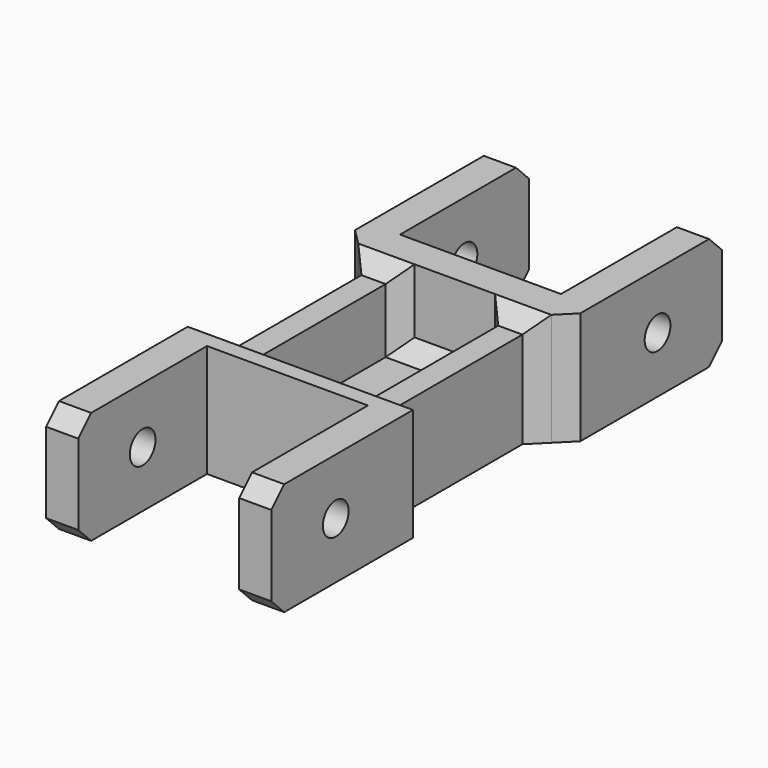
from build123d import *

# Parameters (mm, degrees)
F0_W            = 20
F0_H            = 22
F0_H_2          = 4
F0_H_3          = 20.4
F1_DEPTH        = 2
F2_DEPTH        = 10
F3_R            = 2.2
F4_DEPTH        = 30
F5_W            = 20
F5_H            = 12
F5_R            = 2.6
F7_DEPTH        = 4
F6_W            = 20
F6_H            = 12
F6_R            = 2.6
F8_DEPTH        = 4
F9_T1_DEPTH     = 25
F9_T3_DEPTH     = 57.4
F9_T5_DEPTH     = 16
F9_T7_DEPTH     = 48.4
F9_T9_DEPTH     = 2
F9_T11_DEPTH    = 20
F9_T13_DEPTH    = 7
F9_T15_DEPTH    = 25
F9_T17_DEPTH    = 14
F9_T19_DEPTH    = 27
F9_T21_DEPTH    = 14
F9_T23_DEPTH    = 30
F9_T25_DEPTH    = 7
F9_T27_DEPTH    = 8
F9_S31_W        = 2
F9_S31_H        = 2
F9_T32_DEPTH    = 2
F9_S37_W        = 2
F9_S37_H        = 2
F9_T38_DEPTH    = 2
F9_S43_W        = 2
F9_S43_H        = 2
F9_T44_DEPTH    = 2
F9_S49_W        = 2
F9_S49_H        = 2
F9_T50_DEPTH    = 2
F9_S55_W        = 2
F9_S55_H        = 2
F9_T56_DEPTH    = 2
F9_S61_W        = 2
F9_S61_H        = 2
F9_T62_DEPTH    = 2
F9_S67_W        = 2
F9_S67_H        = 2
F9_T68_DEPTH    = 2
F9_S73_W        = 2
F9_S73_H        = 2
F9_T74_DEPTH    = 2
F9_T81_DEPTH    = 30
F9_T85_DEPTH    = 30
F9_T92_DEPTH    = 7
F9_T96_DEPTH    = 53.4
F9_T103_DEPTH   = 30
F9_T107_DEPTH   = 30
F9_S1_T1_DEPTH  = 7
F9_S1_T3_DEPTH  = 30
F9_S1_T5_DEPTH  = 16
F9_S1_T7_DEPTH  = 8
F9_S1_S11_W     = 2
F9_S1_S11_H     = 2
F9_S1_T12_DEPTH = 2
F9_S1_S17_W     = 2
F9_S1_S17_H     = 2
F9_S1_T18_DEPTH = 2
F9_S1_S23_W     = 2
F9_S1_S23_H     = 2
F9_S1_T24_DEPTH = 2
F9_S1_S29_W     = 2
F9_S1_S29_H     = 2
F9_S1_T30_DEPTH = 2
F10_W           = 20
F10_H           = 30
F11_DEPTH       = 4
F12_W           = 20
F12_H           = 4
F13_DEPTH       = 10
F16_DEPTH       = 4
F17_DEPTH       = 4
F19_W           = 4
F19_H           = 14
F20_DEPTH       = 20
F18_W           = 4
F18_H           = 14
F21_DEPTH       = 20
F22_W           = 22
F22_H           = 8
F23_DEPTH       = 3
F24_W           = 22
F24_H           = 8
F25_DEPTH       = 3
F26_R           = 2
F27_R           = 2
F28_DEPTH       = 28.3421242009
F29_SIZE        = 1.99999


# Not quite as in the source:
# - a fillet or chamfer that OpenCascade refuses, or shapes differently, is made with other operations: its cross-section is extruded or revolved along the edge and cut away or added
# - a fillet or chamfer is up to 0.001 mm smaller than in the source, because OpenCascade refuses the exact size
# - a feature names something its author has since deleted; it is built from what else it names


with BuildPart() as f1:
    # F0 (on Top) → F1 (new body)
    with BuildSketch(Plane.XY):
        with Locations((-44.4073281825, 48.6883277684)):
            Rectangle(F0_W, F0_H)
        with Locations((-44.4073281825, 61.6883277684)):
            Rectangle(F0_W, F0_H_2)
        with Locations((-44.4073281825, 35.6883277684)):
            Rectangle(F0_W, F0_H_2)
        with Locations((-44.4073281825, 23.4883277684)):
            Rectangle(F0_W, F0_H_3)
        with Locations((-44.4073281825, 11.2883277684)):
            Rectangle(F0_W, F0_H_2)
    extrude(amount=-F1_DEPTH)

    # F0 (on Top) → F2 (join)
    with BuildSketch(Plane.XY):
        with Locations((-44.4073281825, 35.6883277684)):
            Rectangle(F0_W, F0_H_2)
        with Locations((-44.4073281825, 61.6883277684)):
            Rectangle(F0_W, F0_H_2)
        with Locations((-44.4073281825, 11.2883277684)):
            Rectangle(F0_W, F0_H_2)
    extrude(amount=F2_DEPTH)

    # F3 (on face) → F4 (cut)
    with BuildSketch(Plane.XZ.offset(-9.2883277684)):
        with Locations((-44.4073281825, 5.5)):
            Circle(F3_R)
    extrude(amount=-F4_DEPTH, mode=Mode.SUBTRACT)

    # F5 (on face) → F7 (join)
    with BuildSketch(Plane(origin=(-54.4073281825, 0, 0), x_dir=(0, -1, 0), z_dir=(-1, 0, 0))):
        with Locations((-73.6883277684, 4)):
            Rectangle(F5_W, F5_H)
        with Locations((-73.6883277684, 4)):
            Circle(F5_R, mode=Mode.SUBTRACT)
    extrude(amount=F7_DEPTH)

    # F6 (on face) → F8 (join)
    with BuildSketch(Plane.YZ.offset(-34.4073281825)):
        with Locations((73.6883277684, 4)):
            Rectangle(F6_W, F6_H)
        with Locations((73.6883277684, 4)):
            Circle(F6_R, mode=Mode.SUBTRACT)
        Polygon((63.6883277684, 10), (59.6883277684, 10), (59.6883277684, 0), (59.6883277684, -2), (63.6883277684, -2), align=None)
    extrude(amount=F8_DEPTH)

    # F9: fillet of radius 2 on 26 edges, made by hand

    # F9_s2 → F9_t1 (cut)
    with BuildSketch(Plane.YZ.offset(-59.4073281825)):
        with BuildLine():
            ThreePointArc((63.6883277684, 0), (63.1025413308, -1.4142135624), (61.6883277684, -2))
            Line((61.6883277684, -2), (63.6883277684, -2))
            Line((63.6883277684, -2), (63.6883277684, 0))
        make_face()
        with BuildLine():
            ThreePointArc((63.6883277684, 8), (63.1025413308, 9.4142135624), (61.6883277684, 10))
            Line((61.6883277684, 10), (63.6883277684, 10))
            Line((63.6883277684, 10), (63.6883277684, 8))
        make_face()
    extrude(amount=F9_T1_DEPTH, mode=Mode.SUBTRACT)

    # F9_s4 → F9_t3 (cut)
    with BuildSketch(Plane.XZ.offset(-68.6883277684)):
        with BuildLine():
            ThreePointArc((-54.4073281825, 0), (-53.8215417448, -1.4142135624), (-52.4073281825, -2))
            Line((-52.4073281825, -2), (-54.4073281825, -2))
            Line((-54.4073281825, -2), (-54.4073281825, 0))
        make_face()
    extrude(amount=F9_T3_DEPTH, mode=Mode.SUBTRACT)

    # F9_s6 → F9_t5 (cut)
    with BuildSketch(Plane.YZ.offset(-52.4073281825)):
        with BuildLine():
            ThreePointArc((9.2883277684, 0), (9.8741142061, -1.4142135624), (11.2883277684, -2))
            Line((11.2883277684, -2), (9.2883277684, -2))
            Line((9.2883277684, -2), (9.2883277684, 0))
        make_face()
        with BuildLine():
            ThreePointArc((9.2883277684, 8), (9.8741142061, 9.4142135624), (11.2883277684, 10))
            Line((11.2883277684, 10), (9.2883277684, 10))
            Line((9.2883277684, 10), (9.2883277684, 8))
        make_face()
    extrude(amount=F9_T5_DEPTH, mode=Mode.SUBTRACT)

    # F9_s8 → F9_t7 (cut)
    with BuildSketch(Plane.XZ.offset(-59.6883277684)):
        with BuildLine():
            ThreePointArc((-34.4073281825, 0), (-34.9931146201, -1.4142135624), (-36.4073281825, -2))
            Line((-36.4073281825, -2), (-34.4073281825, -2))
            Line((-34.4073281825, -2), (-34.4073281825, 0))
        make_face()
    extrude(amount=F9_T7_DEPTH, mode=Mode.SUBTRACT)

    # F9_s10 → F9_t9 (cut)
    with BuildSketch(Plane.YZ.offset(-34.4073281825)):
        with BuildLine():
            ThreePointArc((59.6883277684, 0), (60.2741142061, -1.4142135624), (61.6883277684, -2))
            Line((61.6883277684, -2), (59.6883277684, -2))
            Line((59.6883277684, -2), (59.6883277684, 0))
        make_face()
    extrude(amount=F9_T9_DEPTH, mode=Mode.SUBTRACT)

    # F9_s12 → F9_t11 (cut)
    with BuildSketch(Plane.XZ.offset(-81.6883277684)):
        with BuildLine():
            ThreePointArc((-30.4073281825, 0), (-30.9931146201, -1.4142135624), (-32.4073281825, -2))
            Line((-32.4073281825, -2), (-30.4073281825, -2))
            Line((-30.4073281825, -2), (-30.4073281825, 0))
        make_face()
        with BuildLine():
            ThreePointArc((-30.4073281825, 8), (-30.9931146201, 9.4142135624), (-32.4073281825, 10))
            Line((-32.4073281825, 10), (-30.4073281825, 10))
            Line((-30.4073281825, 10), (-30.4073281825, 8))
        make_face()
    extrude(amount=F9_T11_DEPTH, mode=Mode.SUBTRACT)

    # F9_s14 → F9_t13 (cut)
    with BuildSketch(Plane.YZ.offset(-39.4073281825)):
        with BuildLine():
            ThreePointArc((83.6883277684, 0), (83.1025413308, -1.4142135624), (81.6883277684, -2))
            Line((81.6883277684, -2), (83.6883277684, -2))
            Line((83.6883277684, -2), (83.6883277684, 0))
        make_face()
        with BuildLine():
            ThreePointArc((83.6883277684, 8), (83.1025413308, 9.4142135624), (81.6883277684, 10))
            Line((81.6883277684, 10), (83.6883277684, 10))
            Line((83.6883277684, 10), (83.6883277684, 8))
        make_face()
    extrude(amount=F9_T13_DEPTH, mode=Mode.SUBTRACT)

    # F9_s16 → F9_t15 (cut)
    with BuildSketch(Plane.XZ.offset(-88.6883277684)):
        with BuildLine():
            ThreePointArc((-34.4073281825, 0), (-33.8215417448, -1.4142135624), (-32.4073281825, -2))
            Line((-32.4073281825, -2), (-34.4073281825, -2))
            Line((-34.4073281825, -2), (-34.4073281825, 0))
        make_face()
        with BuildLine():
            ThreePointArc((-34.4073281825, 8), (-33.8215417448, 9.4142135624), (-32.4073281825, 10))
            Line((-32.4073281825, 10), (-34.4073281825, 10))
            Line((-34.4073281825, 10), (-34.4073281825, 8))
        make_face()
    extrude(amount=F9_T15_DEPTH, mode=Mode.SUBTRACT)

    # F9_s18 → F9_t17 (cut)
    with BuildSketch(Plane.XZ.offset(-68.6883277684)):
        with BuildLine():
            ThreePointArc((-52.4073281825, 10), (-53.8215417448, 9.4142135624), (-54.4073281825, 8))
            Line((-54.4073281825, 8), (-54.4073281825, 10))
            Line((-54.4073281825, 10), (-52.4073281825, 10))
        make_face()
    extrude(amount=F9_T17_DEPTH, mode=Mode.SUBTRACT)

    # F9_s20 → F9_t19 (cut)
    with BuildSketch(Plane.YZ.offset(-59.4073281825)):
        with BuildLine():
            ThreePointArc((59.6883277684, 8), (60.2741142061, 9.4142135624), (61.6883277684, 10))
            Line((61.6883277684, 10), (59.6883277684, 10))
            Line((59.6883277684, 10), (59.6883277684, 8))
        make_face()
    extrude(amount=F9_T19_DEPTH, mode=Mode.SUBTRACT)

    # F9_s22 → F9_t21 (cut)
    with BuildSketch(Plane.XZ.offset(-42.6883277684)):
        with BuildLine():
            ThreePointArc((-52.4073281825, 10), (-53.8215417448, 9.4142135624), (-54.4073281825, 8))
            Line((-54.4073281825, 8), (-54.4073281825, 10))
            Line((-54.4073281825, 10), (-52.4073281825, 10))
        make_face()
        with BuildLine():
            ThreePointArc((-36.4073281825, 10), (-34.9931146201, 9.4142135624), (-34.4073281825, 8))
            Line((-34.4073281825, 8), (-34.4073281825, 10))
            Line((-34.4073281825, 10), (-36.4073281825, 10))
        make_face()
    extrude(amount=F9_T21_DEPTH, mode=Mode.SUBTRACT)

    # F9_s24 → F9_t23 (cut)
    with BuildSketch(Plane.YZ.offset(-59.4073281825)):
        with BuildLine():
            ThreePointArc((33.6883277684, 8), (34.2741142061, 9.4142135624), (35.6883277684, 10))
            Line((35.6883277684, 10), (33.6883277684, 10))
            Line((33.6883277684, 10), (33.6883277684, 8))
        make_face()
        with BuildLine():
            ThreePointArc((37.6883277684, 8), (37.1025413308, 9.4142135624), (35.6883277684, 10))
            Line((35.6883277684, 10), (37.6883277684, 10))
            Line((37.6883277684, 10), (37.6883277684, 8))
        make_face()
        with BuildLine():
            ThreePointArc((13.2883277684, 8), (12.7025413308, 9.4142135624), (11.2883277684, 10))
            Line((11.2883277684, 10), (13.2883277684, 10))
            Line((13.2883277684, 10), (13.2883277684, 8))
        make_face()
    extrude(amount=F9_T23_DEPTH, mode=Mode.SUBTRACT)

    # F9_s26 → F9_t25 (cut)
    with BuildSketch(Plane.XZ.offset(-18.2883277684)):
        with BuildLine():
            ThreePointArc((-36.4073281825, 10), (-34.9931146201, 9.4142135624), (-34.4073281825, 8))
            Line((-34.4073281825, 8), (-34.4073281825, 10))
            Line((-34.4073281825, 10), (-36.4073281825, 10))
        make_face()
        with BuildLine():
            ThreePointArc((-52.4073281825, 10), (-53.8215417448, 9.4142135624), (-54.4073281825, 8))
            Line((-54.4073281825, 8), (-54.4073281825, 10))
            Line((-54.4073281825, 10), (-52.4073281825, 10))
        make_face()
    extrude(amount=F9_T25_DEPTH, mode=Mode.SUBTRACT)

    # F9_s28 → F9_t27 (cut)
    with BuildSketch(Plane.XY):
        with BuildLine():
            ThreePointArc((-36.4073281825, 9.2883277684), (-34.9931146201, 9.8741142061), (-34.4073281825, 11.2883277684))
            Line((-34.4073281825, 11.2883277684), (-34.4073281825, 9.2883277684))
            Line((-34.4073281825, 9.2883277684), (-36.4073281825, 9.2883277684))
        make_face()
        with BuildLine():
            ThreePointArc((-52.4073281825, 9.2883277684), (-53.8215417448, 9.8741142061), (-54.4073281825, 11.2883277684))
            Line((-54.4073281825, 11.2883277684), (-54.4073281825, 9.2883277684))
            Line((-54.4073281825, 9.2883277684), (-52.4073281825, 9.2883277684))
        make_face()
        with BuildLine():
            ThreePointArc((-30.4073281825, 61.6883277684), (-30.9931146201, 60.2741142061), (-32.4073281825, 59.6883277684))
            Line((-32.4073281825, 59.6883277684), (-30.4073281825, 59.6883277684))
            Line((-30.4073281825, 59.6883277684), (-30.4073281825, 61.6883277684))
        make_face()
        with BuildLine():
            ThreePointArc((-30.4073281825, 81.6883277684), (-30.9931146201, 83.1025413308), (-32.4073281825, 83.6883277684))
            Line((-32.4073281825, 83.6883277684), (-30.4073281825, 83.6883277684))
            Line((-30.4073281825, 83.6883277684), (-30.4073281825, 81.6883277684))
        make_face()
    extrude(amount=F9_T27_DEPTH, mode=Mode.SUBTRACT)


with BuildPart() as f9_tool30:
    # F9_s31 → F9_t32 (new body)
    with BuildSketch(Plane.YZ.offset(-52.4073281825)):
        with Locations((10.2883277684, -1)):
            Rectangle(F9_S31_W, F9_S31_H)
    extrude(amount=-F9_T32_DEPTH)

    # F9_s33 → F9_t34 (revolve, cut)
    with BuildSketch(Plane(origin=(-52.4073281825, 11.2883277684, 0), x_dir=(0, 0.7071067812, 0.7071067812), z_dir=(0, -0.7071067812, 0.7071067812))):
        with BuildLine():
            ThreePointArc((0, -2), (2, 0), (0, 2))
            Line((0, 2), (0, -2))
        make_face()
    revolve(axis=Axis((-52.4073281825, 11.2883277684, 0), (-1, 0, 0)), mode=Mode.SUBTRACT)


with BuildPart() as f1_1:
    add(f1.part)

    # F9_t29: cut F9_tool30
    add(f9_tool30.part, mode=Mode.SUBTRACT)


with BuildPart() as f9_tool36:
    # F9_s37 → F9_t38 (new body)
    with BuildSketch(Plane.XY):
        with Locations((-35.4073281825, 10.2883277684)):
            Rectangle(F9_S37_W, F9_S37_H)
    extrude(amount=-F9_T38_DEPTH)

    # F9_s39 → F9_t40 (revolve, cut)
    with BuildSketch(Plane(origin=(-36.4073281825, 11.2883277684, 0), x_dir=(-0.7071067812, 0.7071067812, 0), z_dir=(-0.7071067812, -0.7071067812, 0))):
        with BuildLine():
            ThreePointArc((0, -2), (2, 0), (0, 2))
            Line((0, 2), (0, -2))
        make_face()
    revolve(axis=Axis((-36.4073281825, 11.2883277684, 0), (0, 0, -1)), mode=Mode.SUBTRACT)


with BuildPart() as f1_2:
    add(f1_1.part)

    # F9_t35: cut F9_tool36
    add(f9_tool36.part, mode=Mode.SUBTRACT)


with BuildPart() as f9_tool42:
    # F9_s43 → F9_t44 (new body)
    with BuildSketch(Plane.YZ.offset(-32.4073281825)):
        with Locations((60.6883277684, -1)):
            Rectangle(F9_S43_W, F9_S43_H)
    extrude(amount=F9_T44_DEPTH)

    # F9_s45 → F9_t46 (revolve, cut)
    with BuildSketch(Plane(origin=(-32.4073281825, 61.6883277684, 0), x_dir=(0, 0.7071067812, 0.7071067812), z_dir=(0, 0.7071067812, -0.7071067812))):
        with BuildLine():
            ThreePointArc((0, -2), (2, 0), (0, 2))
            Line((0, 2), (0, -2))
        make_face()
    revolve(axis=Axis((-32.4073281825, 61.6883277684, 0), (1, 0, 0)), mode=Mode.SUBTRACT)


with BuildPart() as f1_3:
    add(f1_2.part)

    # F9_t41: cut F9_tool42
    add(f9_tool42.part, mode=Mode.SUBTRACT)


with BuildPart() as f9_tool48:
    # F9_s49 → F9_t50 (new body)
    with BuildSketch(Plane.XY):
        with Locations((-31.4073281825, 82.6883277684)):
            Rectangle(F9_S49_W, F9_S49_H)
    extrude(amount=-F9_T50_DEPTH)

    # F9_s51 → F9_t52 (revolve, cut)
    with BuildSketch(Plane(origin=(-32.4073281825, 81.6883277684, 0), x_dir=(-0.7071067812, -0.7071067812, 0), z_dir=(0.7071067812, -0.7071067812, 0))):
        with BuildLine():
            ThreePointArc((0, -2), (2, 0), (0, 2))
            Line((0, 2), (0, -2))
        make_face()
    revolve(axis=Axis((-32.4073281825, 81.6883277684, 0), (0, 0, -1)), mode=Mode.SUBTRACT)


with BuildPart() as f1_4:
    add(f1_3.part)

    # F9_t47: cut F9_tool48
    add(f9_tool48.part, mode=Mode.SUBTRACT)


with BuildPart() as f9_tool54:
    # F9_s55 → F9_t56 (new body)
    with BuildSketch(Plane.XY.offset(8)):
        with Locations((-31.4073281825, 60.6883277684)):
            Rectangle(F9_S55_W, F9_S55_H)
    extrude(amount=F9_T56_DEPTH)

    # F9_s57 → F9_t58 (revolve, cut)
    with BuildSketch(Plane(origin=(-32.4073281825, 61.6883277684, 8), x_dir=(-0.7071067812, 0.7071067812, 0), z_dir=(0.7071067812, 0.7071067812, 0))):
        with BuildLine():
            ThreePointArc((0, -2), (2, 0), (0, 2))
            Line((0, 2), (0, -2))
        make_face()
    revolve(axis=Axis((-32.4073281825, 61.6883277684, 8), (0, 0, 1)), mode=Mode.SUBTRACT)


with BuildPart() as f1_5:
    add(f1_4.part)

    # F9_t53: cut F9_tool54
    add(f9_tool54.part, mode=Mode.SUBTRACT)


with BuildPart() as f9_tool60:
    # F9_s61 → F9_t62 (new body)
    with BuildSketch(Plane.XZ.offset(-81.6883277684)):
        with Locations((-31.4073281825, 9)):
            Rectangle(F9_S61_W, F9_S61_H)
    extrude(amount=-F9_T62_DEPTH)

    # F9_s63 → F9_t64 (revolve, cut)
    with BuildSketch(Plane(origin=(-32.4073281825, 81.6883277684, 8), x_dir=(-0.7071067812, 0, -0.7071067812), z_dir=(0.7071067812, 0, -0.7071067812))):
        with BuildLine():
            ThreePointArc((0, -2), (2, 0), (0, 2))
            Line((0, 2), (0, -2))
        make_face()
    revolve(axis=Axis((-32.4073281825, 81.6883277684, 8), (0, 1, 0)), mode=Mode.SUBTRACT)


with BuildPart() as f1_6:
    add(f1_5.part)

    # F9_t59: cut F9_tool60
    add(f9_tool60.part, mode=Mode.SUBTRACT)


with BuildPart() as f9_tool66:
    # F9_s67 → F9_t68 (new body)
    with BuildSketch(Plane.XZ.offset(-11.2883277684)):
        with Locations((-35.4073281825, 9)):
            Rectangle(F9_S67_W, F9_S67_H)
    extrude(amount=F9_T68_DEPTH)

    # F9_s69 → F9_t70 (revolve, cut)
    with BuildSketch(Plane(origin=(-36.4073281825, 11.2883277684, 8), x_dir=(-0.7071067812, 0, -0.7071067812), z_dir=(-0.7071067812, 0, 0.7071067812))):
        with BuildLine():
            ThreePointArc((0, -2), (2, 0), (0, 2))
            Line((0, 2), (0, -2))
        make_face()
    revolve(axis=Axis((-36.4073281825, 11.2883277684, 8), (0, -1, 0)), mode=Mode.SUBTRACT)


with BuildPart() as f1_7:
    add(f1_6.part)

    # F9_t65: cut F9_tool66
    add(f9_tool66.part, mode=Mode.SUBTRACT)


with BuildPart() as f9_tool72:
    # F9_s73 → F9_t74 (new body)
    with BuildSketch(Plane.YZ.offset(-52.4073281825)):
        with Locations((10.2883277684, 9)):
            Rectangle(F9_S73_W, F9_S73_H)
    extrude(amount=-F9_T74_DEPTH)

    # F9_s75 → F9_t76 (revolve, cut)
    with BuildSketch(Plane(origin=(-52.4073281825, 11.2883277684, 8), x_dir=(0, 0.7071067812, -0.7071067812), z_dir=(0, 0.7071067812, 0.7071067812))):
        with BuildLine():
            ThreePointArc((0, -2), (2, 0), (0, 2))
            Line((0, 2), (0, -2))
        make_face()
    revolve(axis=Axis((-52.4073281825, 11.2883277684, 8), (-1, 0, 0)), mode=Mode.SUBTRACT)


with BuildPart() as f1_8:
    add(f1_7.part)

    # F9_t71: cut F9_tool72
    add(f9_tool72.part, mode=Mode.SUBTRACT)


with BuildPart() as f9_tool79:
    # F9_s80 → F9_t81 (new body)
    with BuildSketch(Plane.YZ.offset(-29.4073281825)):
        with BuildLine():
            ThreePointArc((63.6883277684, 0), (63.1025413308, -1.4142135624), (61.6883277684, -2))
            Line((61.6883277684, -2), (63.6883277684, -2))
            Line((63.6883277684, -2), (63.6883277684, 0))
        make_face()
    extrude(amount=-F9_T81_DEPTH)

    split(bisect_by=Plane.YZ.offset(-34.4073281825), keep=Keep.TOP)


with BuildPart() as f9_tool83:
    # F9_s84 → F9_t85 (new body)
    with BuildSketch(Plane.XZ.offset(-58.6883277684)):
        with BuildLine():
            ThreePointArc((-34.4073281825, 0), (-33.8215417448, -1.4142135624), (-32.4073281825, -2))
            Line((-32.4073281825, -2), (-34.4073281825, -2))
            Line((-34.4073281825, -2), (-34.4073281825, 0))
        make_face()
    extrude(amount=-F9_T85_DEPTH)

    split(bisect_by=Plane.XZ.offset(-63.6883277684), keep=Keep.TOP)


with BuildPart() as f9_tool79_1:
    add(f9_tool79.part)

    # F9_t87: intersect F9_tool83
    add(f9_tool83.part, mode=Mode.INTERSECT)


with BuildPart() as f1_9:
    add(f1_8.part)

    # F9_t77: cut F9_tool79
    add(f9_tool79_1.part, mode=Mode.SUBTRACT)


with BuildPart() as f9_tool90:
    # F9_s91 → F9_t92 (new body)
    with BuildSketch(Plane.YZ.offset(-39.4073281825)):
        with BuildLine():
            ThreePointArc((59.6883277684, 0), (60.2741142061, -1.4142135624), (61.6883277684, -2))
            Line((61.6883277684, -2), (59.6883277684, -2))
            Line((59.6883277684, -2), (59.6883277684, 0))
        make_face()
    extrude(amount=F9_T92_DEPTH)

    split(bisect_by=Plane.YZ.offset(-34.4073281825), keep=Keep.BOTTOM)


with BuildPart() as f9_tool94:
    # F9_s95 → F9_t96 (new body)
    with BuildSketch(Plane.XZ.offset(-11.2883277684)):
        with BuildLine():
            ThreePointArc((-34.4073281825, 0), (-34.9931146201, -1.4142135624), (-36.4073281825, -2))
            Line((-36.4073281825, -2), (-34.4073281825, -2))
            Line((-34.4073281825, -2), (-34.4073281825, 0))
        make_face()
    extrude(amount=-F9_T96_DEPTH)

    split(bisect_by=Plane.XZ.offset(-59.6883277684), keep=Keep.BOTTOM)


with BuildPart() as f9_tool90_1:
    add(f9_tool90.part)

    # F9_t98: intersect F9_tool94
    add(f9_tool94.part, mode=Mode.INTERSECT)


with BuildPart() as f1_10:
    add(f1_9.part)

    # F9_t88: cut F9_tool90
    add(f9_tool90_1.part, mode=Mode.SUBTRACT)


with BuildPart() as f9_tool101:
    # F9_s102 → F9_t103 (new body)
    with BuildSketch(Plane.YZ.offset(-29.4073281825)):
        with BuildLine():
            ThreePointArc((63.6883277684, 8), (63.1025413308, 9.4142135624), (61.6883277684, 10))
            Line((61.6883277684, 10), (63.6883277684, 10))
            Line((63.6883277684, 10), (63.6883277684, 8))
        make_face()
    extrude(amount=-F9_T103_DEPTH)

    split(bisect_by=Plane.YZ.offset(-34.4073281825), keep=Keep.TOP)


with BuildPart() as f9_tool105:
    # F9_s106 → F9_t107 (new body)
    with BuildSketch(Plane.XZ.offset(-88.6883277684)):
        with BuildLine():
            ThreePointArc((-34.4073281825, 8), (-33.8215417448, 9.4142135624), (-32.4073281825, 10))
            Line((-32.4073281825, 10), (-34.4073281825, 10))
            Line((-34.4073281825, 10), (-34.4073281825, 8))
        make_face()
    extrude(amount=F9_T107_DEPTH)

    split(bisect_by=Plane.XZ.offset(-63.6883277684), keep=Keep.TOP)


with BuildPart() as f9_tool101_1:
    add(f9_tool101.part)

    # F9_t109: intersect F9_tool105
    add(f9_tool105.part, mode=Mode.INTERSECT)


with BuildPart() as f1_11:
    add(f1_10.part)

    # F9_t99: cut F9_tool101
    add(f9_tool101_1.part, mode=Mode.SUBTRACT)

    # F9#s1: fillet of radius 2 on 10 edges, made by hand

    # F9_s1_s2 → F9_s1_t1 (cut)
    with BuildSketch(Plane.YZ.offset(-56.4073281825)):
        with BuildLine():
            ThreePointArc((83.6883277684, 0), (83.1025413308, -1.4142135624), (81.6883277684, -2))
            Line((81.6883277684, -2), (83.6883277684, -2))
            Line((83.6883277684, -2), (83.6883277684, 0))
        make_face()
        with BuildLine():
            ThreePointArc((63.6883277684, 0), (64.2741142061, -1.4142135624), (65.6883277684, -2))
            Line((65.6883277684, -2), (63.6883277684, -2))
            Line((63.6883277684, -2), (63.6883277684, 0))
        make_face()
        with BuildLine():
            ThreePointArc((63.6883277684, 8), (64.2741142061, 9.4142135624), (65.6883277684, 10))
            Line((65.6883277684, 10), (63.6883277684, 10))
            Line((63.6883277684, 10), (63.6883277684, 8))
        make_face()
        with BuildLine():
            ThreePointArc((81.6883277684, 10), (83.1025413308, 9.4142135624), (83.6883277684, 8))
            Line((83.6883277684, 8), (83.6883277684, 10))
            Line((83.6883277684, 10), (81.6883277684, 10))
        make_face()
    extrude(amount=F9_S1_T1_DEPTH, mode=Mode.SUBTRACT)

    # F9_s1_s4 → F9_s1_t3 (cut)
    with BuildSketch(Plane.XZ.offset(-88.6883277684)):
        with BuildLine():
            ThreePointArc((-56.4073281825, -2), (-54.9931146201, -1.4142135624), (-54.4073281825, 0))
            Line((-54.4073281825, 0), (-54.4073281825, -2))
            Line((-54.4073281825, -2), (-56.4073281825, -2))
        make_face()
        with BuildLine():
            ThreePointArc((-56.4073281825, 10), (-54.9931146201, 9.4142135624), (-54.4073281825, 8))
            Line((-54.4073281825, 8), (-54.4073281825, 10))
            Line((-54.4073281825, 10), (-56.4073281825, 10))
        make_face()
    extrude(amount=F9_S1_T3_DEPTH, mode=Mode.SUBTRACT)

    # F9_s1_s6 → F9_s1_t5 (cut)
    with BuildSketch(Plane.XZ.offset(-81.6883277684)):
        with BuildLine():
            ThreePointArc((-58.4073281825, 0), (-57.8215417448, -1.4142135624), (-56.4073281825, -2))
            Line((-56.4073281825, -2), (-58.4073281825, -2))
            Line((-58.4073281825, -2), (-58.4073281825, 0))
        make_face()
        with BuildLine():
            ThreePointArc((-56.4073281825, 10), (-57.8215417448, 9.4142135624), (-58.4073281825, 8))
            Line((-58.4073281825, 8), (-58.4073281825, 10))
            Line((-58.4073281825, 10), (-56.4073281825, 10))
        make_face()
    extrude(amount=F9_S1_T5_DEPTH, mode=Mode.SUBTRACT)

    # F9_s1_s8 → F9_s1_t7 (cut)
    with BuildSketch(Plane.XY):
        with BuildLine():
            ThreePointArc((-56.4073281825, 63.6883277684), (-57.8215417448, 64.2741142061), (-58.4073281825, 65.6883277684))
            Line((-58.4073281825, 65.6883277684), (-58.4073281825, 63.6883277684))
            Line((-58.4073281825, 63.6883277684), (-56.4073281825, 63.6883277684))
        make_face()
        with BuildLine():
            ThreePointArc((-56.4073281825, 83.6883277684), (-57.8215417448, 83.1025413308), (-58.4073281825, 81.6883277684))
            Line((-58.4073281825, 81.6883277684), (-58.4073281825, 83.6883277684))
            Line((-58.4073281825, 83.6883277684), (-56.4073281825, 83.6883277684))
        make_face()
    extrude(amount=F9_S1_T7_DEPTH, mode=Mode.SUBTRACT)


with BuildPart() as f9_s1_tool10:
    # F9_s1_s11 → F9_s1_t12 (new body)
    with BuildSketch(Plane.XZ.offset(-81.6883277684)):
        with Locations((-57.4073281825, -1)):
            Rectangle(F9_S1_S11_W, F9_S1_S11_H)
    extrude(amount=-F9_S1_T12_DEPTH)

    # F9_s1_s13 → F9_s1_t14 (revolve, cut)
    with BuildSketch(Plane(origin=(-56.4073281825, 81.6883277684, 0), x_dir=(0.7071067812, 0, 0.7071067812), z_dir=(-0.7071067812, 0, 0.7071067812))):
        with BuildLine():
            ThreePointArc((0, -2), (2, 0), (0, 2))
            Line((0, 2), (0, -2))
        make_face()
    revolve(axis=Axis((-56.4073281825, 81.6883277684, 0), (0, 1, 0)), mode=Mode.SUBTRACT)


with BuildPart() as f1_12:
    add(f1_11.part)

    # F9_s1_t9: cut F9_s1_tool10
    add(f9_s1_tool10.part, mode=Mode.SUBTRACT)


with BuildPart() as f9_s1_tool16:
    # F9_s1_s17 → F9_s1_t18 (new body)
    with BuildSketch(Plane.XZ.offset(-65.6883277684)):
        with Locations((-57.4073281825, -1)):
            Rectangle(F9_S1_S17_W, F9_S1_S17_H)
    extrude(amount=F9_S1_T18_DEPTH)

    # F9_s1_s19 → F9_s1_t20 (revolve, cut)
    with BuildSketch(Plane(origin=(-56.4073281825, 65.6883277684, 0), x_dir=(0.7071067812, 0, 0.7071067812), z_dir=(0.7071067812, 0, -0.7071067812))):
        with BuildLine():
            ThreePointArc((0, -2), (2, 0), (0, 2))
            Line((0, 2), (0, -2))
        make_face()
    revolve(axis=Axis((-56.4073281825, 65.6883277684, 0), (0, -1, 0)), mode=Mode.SUBTRACT)


with BuildPart() as f1_13:
    add(f1_12.part)

    # F9_s1_t15: cut F9_s1_tool16
    add(f9_s1_tool16.part, mode=Mode.SUBTRACT)


with BuildPart() as f9_s1_tool22:
    # F9_s1_s23 → F9_s1_t24 (new body)
    with BuildSketch(Plane.XZ.offset(-65.6883277684)):
        with Locations((-57.4073281825, 9)):
            Rectangle(F9_S1_S23_W, F9_S1_S23_H)
    extrude(amount=F9_S1_T24_DEPTH)

    # F9_s1_s25 → F9_s1_t26 (revolve, cut)
    with BuildSketch(Plane(origin=(-56.4073281825, 65.6883277684, 8), x_dir=(0.7071067812, 0, -0.7071067812), z_dir=(-0.7071067812, 0, -0.7071067812))):
        with BuildLine():
            ThreePointArc((0, -2), (2, 0), (0, 2))
            Line((0, 2), (0, -2))
        make_face()
    revolve(axis=Axis((-56.4073281825, 65.6883277684, 8), (0, -1, 0)), mode=Mode.SUBTRACT)


with BuildPart() as f1_14:
    add(f1_13.part)

    # F9_s1_t21: cut F9_s1_tool22
    add(f9_s1_tool22.part, mode=Mode.SUBTRACT)


with BuildPart() as f9_s1_tool28:
    # F9_s1_s29 → F9_s1_t30 (new body)
    with BuildSketch(Plane.XY.offset(8)):
        with Locations((-57.4073281825, 82.6883277684)):
            Rectangle(F9_S1_S29_W, F9_S1_S29_H)
    extrude(amount=F9_S1_T30_DEPTH)

    # F9_s1_s31 → F9_s1_t32 (revolve, cut)
    with BuildSketch(Plane(origin=(-56.4073281825, 81.6883277684, 8), x_dir=(0.7071067812, -0.7071067812, 0), z_dir=(-0.7071067812, -0.7071067812, 0))):
        with BuildLine():
            ThreePointArc((0, -2), (2, 0), (0, 2))
            Line((0, 2), (0, -2))
        make_face()
    revolve(axis=Axis((-56.4073281825, 81.6883277684, 8), (0, 0, 1)), mode=Mode.SUBTRACT)


with BuildPart() as f1_15:
    add(f1_14.part)

    # F9_s1_t27: cut F9_s1_tool28
    add(f9_s1_tool28.part, mode=Mode.SUBTRACT)


with BuildPart() as f11:
    # F10 (on Top) → F11 (new body)
    with BuildSketch(Plane.XY):
        with Locations((-44.0662039816, -66.8389573097)):
            Rectangle(F10_W, F10_H)
    extrude(amount=F11_DEPTH)

    # F12 (on face) → F13 (join)
    with BuildSketch(Plane.XY.offset(4)):
        with Locations((-44.0662039816, -53.8389573097)):
            Rectangle(F12_W, F12_H)
        with Locations((-44.0662039816, -79.8389573097)):
            Rectangle(F12_W, F12_H)
    extrude(amount=F13_DEPTH)

    # F15 (on face) → F16 (join)
    with BuildSketch(Plane.YZ.offset(-34.0662039816)):
        Polygon((-77.8389573097, 0), (-77.8389573097, 4), (-77.8389573097, 14), (-81.8389573097, 14), (-81.8389573097, 0), align=None)
        Polygon((-55.8389573097, 14), (-55.8389573097, 4), (-55.8389573097, 0), (-51.8389573097, 0), (-51.8389573097, 14), align=None)
    extrude(amount=F16_DEPTH)

    # F14 (on face) → F17 (join)
    with BuildSketch(Plane(origin=(-54.0662039816, 0, 0), x_dir=(0, -1, 0), z_dir=(-1, 0, 0))):
        Polygon((55.8389573097, 0), (55.8389573097, 4), (55.8389573097, 14), (51.8389573097, 14), (51.8389573097, 0), align=None)
        Polygon((77.8389573097, 14), (77.8389573097, 4), (77.8389573097, 0), (81.8389573097, 0), (81.8389573097, 14), align=None)
    extrude(amount=F17_DEPTH)

    # F19 (on face) → F20 (join)
    with BuildSketch(Plane.XZ.offset(81.8389573097)):
        with Locations((-56.0662039816, 7)):
            Rectangle(F19_W, F19_H)
        with Locations((-32.0662039816, 7)):
            Rectangle(F19_W, F19_H)
    extrude(amount=F20_DEPTH)

    # F18 (on face) → F21 (join)
    with BuildSketch(Plane(origin=(0, -51.8389573097, 0), x_dir=(-1, 0, 0), z_dir=(0, 1, 0))):
        with Locations((32.0662039816, 7)):
            Rectangle(F18_W, F18_H)
        with Locations((56.0662039816, 7)):
            Rectangle(F18_W, F18_H)
    extrude(amount=F21_DEPTH)

    # F22 (on face) → F23 (join)
    with BuildSketch(Plane(origin=(-54.0662039816, 0, 0), x_dir=(0, -1, 0), z_dir=(-1, 0, 0))):
        with Locations((66.8389573097, 8)):
            Rectangle(F22_W, F22_H)
    extrude(amount=-F23_DEPTH)

    # F24 (on face) → F25 (join)
    with BuildSketch(Plane.YZ.offset(-34.0662039816)):
        with Locations((-66.8389573097, 8)):
            Rectangle(F24_W, F24_H)
    extrude(amount=-F25_DEPTH)

    # F26 (on face) + F27 (on face) → F28 (cut, through all)
    with BuildSketch(Plane.YZ.offset(-30.0662039816)):
        with Locations((-91.8389573097, 7)):
            Circle(F26_R)
    with BuildSketch(Plane.YZ.offset(-30.0662039816)):
        with Locations((-41.8389573097, 7)):
            Circle(F27_R)
    extrude(amount=-F28_DEPTH, mode=Mode.SUBTRACT)

    # F29 (size 2 in the source; OpenCascade refuses exactly that, so slightly less here)
    f29_edges = [f11.edges().sort_by_distance(p)[0] for p in [
        (-32.066204, -101.838957, 0),
        (-30.066204, -77.838957, 7),
        (-44.066204, -77.838957, 4),
        (-44.066204, -77.838957, 14),
        (-58.066204, -77.838957, 7),
        (-44.066204, -55.838957, 4),
        (-51.066204, -55.838957, 8),
        (-37.066204, -55.838957, 8),
        (-34.066204, -55.838957, 6),
        (-35.566204, -55.838957, 12),
        (-52.566204, -55.838957, 12),
        (-54.066204, -55.838957, 6),
        (-30.066204, -55.838957, 7),
        (-58.066204, -55.838957, 7),
        (-32.066204, -31.838957, 14),
        (-56.066204, -31.838957, 14),
        (-56.066204, -31.838957, 0),
        (-32.066204, -31.838957, 0),
        (-56.066204, -101.838957, 14),
        (-32.066204, -101.838957, 14),
        (-56.066204, -101.838957, 0),
    ]]
    chamfer(f29_edges, length=F29_SIZE)


solid = f11.part
